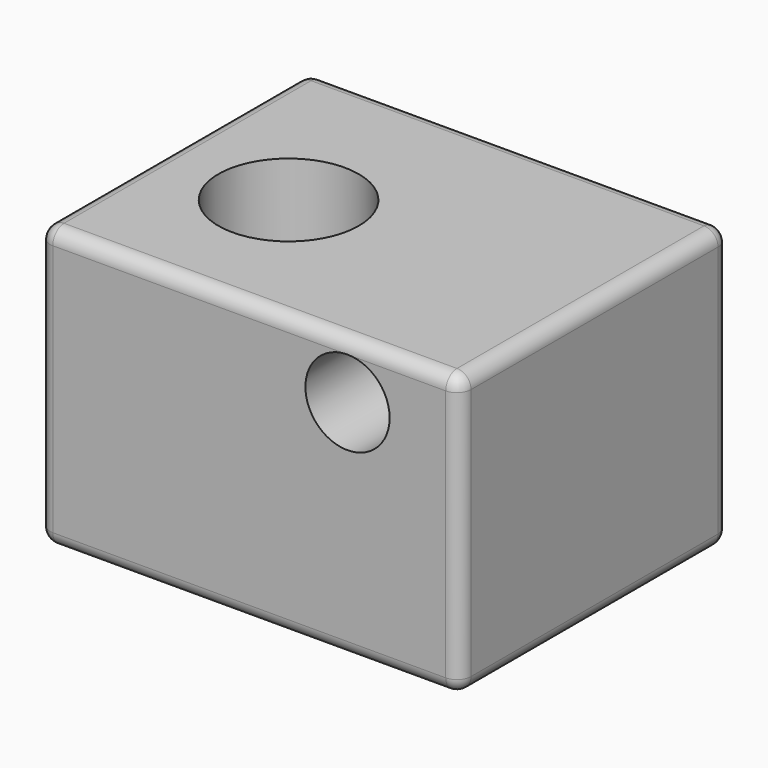
from build123d import *

# Parameters (mm, degrees)
F0_W         = 15
F0_H         = 12
F0_R         = 2.5
F1_DEPTH     = 5
F2_R         = 1.5
F3_DEPTH     = 12.001
F4_R         = 0.49999
F5_T1_DEPTH  = 9.5
F5_T3_DEPTH  = 11
F5_T5_DEPTH  = 14
F5_T8_ANGLE  = 90
F5_T10_ANGLE = 90
F5_T12_ANGLE = 90
F5_T14_ANGLE = 90
F5_S17_W     = 0.5
F5_S17_H     = 0.5
F5_T18_DEPTH = 0.5
F5_S23_W     = 0.5
F5_S23_H     = 0.5
F5_T24_DEPTH = 0.5
F5_S29_W     = 0.5
F5_S29_H     = 0.5
F5_T30_DEPTH = 0.5
F5_S35_W     = 0.5
F5_S35_H     = 0.5
F5_T36_DEPTH = 0.5


# Not quite as in the source:
# - a fillet or chamfer that OpenCascade refuses, or shapes differently, is made with other operations: its cross-section is extruded or revolved along the edge and cut away or added
# - a fillet or chamfer is up to 0.001 mm smaller than in the source, because OpenCascade refuses the exact size


with BuildPart() as f1:
    # F0 (on Top) → F1 (new body, symmetric)
    with BuildSketch(Plane.XY):
        with Locations((7.5, 6)):
            Rectangle(F0_W, F0_H)
        with Locations((4.5, 5.5)):
            Circle(F0_R, mode=Mode.SUBTRACT)
    extrude(amount=F1_DEPTH, both=True)

    # F2 (on face) → F3 (cut, through all)
    with BuildSketch(Plane.XZ):
        with Locations((11, 3)):
            Circle(F2_R)
    extrude(amount=-F3_DEPTH, mode=Mode.SUBTRACT)

    # F4 (radius 0.5 in the source; OpenCascade refuses exactly that, so slightly less here)
    f4_edges = [f1.edges().sort_by_distance(p)[0] for p in [
        (7.5, 0, 5),
        (15, 6, 5),
        (7.5, 12, 5),
        (0, 6, 5),
    ]]
    fillet(f4_edges, radius=F4_R)

    # F5: fillet of radius 0.5 on 8 edges, made by hand

    # F5_s2 → F5_t1 (cut)
    with BuildSketch(Plane.XY.offset(-4.5)):
        with BuildLine():
            ThreePointArc((14.5, 0), (14.8535533906, 0.1464466094), (15, 0.5))
            Line((15, 0.5), (15, 0))
            Line((15, 0), (14.5, 0))
        make_face()
        with BuildLine():
            ThreePointArc((0, 0.5), (0.1464466094, 0.1464466094), (0.5, 0))
            Line((0.5, 0), (0, 0))
            Line((0, 0), (0, 0.5))
        make_face()
        with BuildLine():
            ThreePointArc((0, 11.5), (0.1464466094, 11.8535533906), (0.5, 12))
            Line((0.5, 12), (0, 12))
            Line((0, 12), (0, 11.5))
        make_face()
        with BuildLine():
            ThreePointArc((14.5, 12), (14.8535533906, 11.8535533906), (15, 11.5))
            Line((15, 11.5), (15, 12))
            Line((15, 12), (14.5, 12))
        make_face()
    extrude(amount=F5_T1_DEPTH, mode=Mode.SUBTRACT)

    # F5_s4 → F5_t3 (cut)
    with BuildSketch(Plane.XZ.offset(-11.5)):
        with BuildLine():
            ThreePointArc((0, -4.5), (0.1464466094, -4.8535533906), (0.5, -5))
            Line((0.5, -5), (0, -5))
            Line((0, -5), (0, -4.5))
        make_face()
        with BuildLine():
            ThreePointArc((14.5, -5), (14.8535533906, -4.8535533906), (15, -4.5))
            Line((15, -4.5), (15, -5))
            Line((15, -5), (14.5, -5))
        make_face()
    extrude(amount=F5_T3_DEPTH, mode=Mode.SUBTRACT)

    # F5_s6 → F5_t5 (cut)
    with BuildSketch(Plane.YZ.offset(0.5)):
        with BuildLine():
            ThreePointArc((11.5, -5), (11.8535533906, -4.8535533906), (12, -4.5))
            Line((12, -4.5), (12, -5))
            Line((12, -5), (11.5, -5))
        make_face()
        with BuildLine():
            ThreePointArc((0, -4.5), (0.1464466094, -4.8535533906), (0.5, -5))
            Line((0.5, -5), (0, -5))
            Line((0, -5), (0, -4.5))
        make_face()
    extrude(amount=F5_T5_DEPTH, mode=Mode.SUBTRACT)

    # F5_s7 → F5_t8 (revolve, cut)
    with BuildSketch(Plane.XZ.offset(-11.5)):
        with BuildLine():
            ThreePointArc((14.50001, 5), (14.8535563195, 4.8535563195), (15, 4.50001))
            Line((15, 4.50001), (15, 5))
            Line((15, 5), (14.50001, 5))
        make_face()
    revolve(axis=Axis((14.5, 11.5, 5), (0, 0, 1)), revolution_arc=F5_T8_ANGLE, mode=Mode.SUBTRACT)

    # F5_s9 → F5_t10 (revolve, cut)
    with BuildSketch(Plane.YZ.offset(0.5)):
        with BuildLine():
            ThreePointArc((11.50001, 5), (11.8535563195, 4.8535563195), (12, 4.50001))
            Line((12, 4.50001), (12, 5))
            Line((12, 5), (11.50001, 5))
        make_face()
    revolve(axis=Axis((0.5, 11.5, 5), (0, 0, 1)), revolution_arc=F5_T10_ANGLE, mode=Mode.SUBTRACT)

    # F5_s11 → F5_t12 (revolve, cut)
    with BuildSketch(Plane.XZ.offset(-0.5)):
        with BuildLine():
            ThreePointArc((0.49999, 5), (0.1464436805, 4.8535563195), (0, 4.50001))
            Line((0, 4.50001), (0, 5))
            Line((0, 5), (0.49999, 5))
        make_face()
    revolve(axis=Axis((0.5, 0.5, 5), (0, 0, 1)), revolution_arc=F5_T12_ANGLE, mode=Mode.SUBTRACT)

    # F5_s13 → F5_t14 (revolve, cut)
    with BuildSketch(Plane.YZ.offset(14.5)):
        with BuildLine():
            ThreePointArc((0.49999, 5), (0.1464436805, 4.8535563195), (0, 4.50001))
            Line((0, 4.50001), (0, 5))
            Line((0, 5), (0.49999, 5))
        make_face()
    revolve(axis=Axis((14.5, 0.5, 5), (0, 0, 1)), revolution_arc=F5_T14_ANGLE, mode=Mode.SUBTRACT)


with BuildPart() as f5_tool16:
    # F5_s17 → F5_t18 (new body)
    with BuildSketch(Plane.XZ.offset(-0.5)):
        with Locations((14.75, -4.75)):
            Rectangle(F5_S17_W, F5_S17_H)
    extrude(amount=F5_T18_DEPTH)

    # F5_s19 → F5_t20 (revolve, cut)
    with BuildSketch(Plane(origin=(14.5, 0.5, -4.5), x_dir=(-0.7071067812, 0, 0.7071067812), z_dir=(0.7071067812, 0, 0.7071067812))):
        with BuildLine():
            ThreePointArc((0, -0.5), (0.5, 0), (0, 0.5))
            Line((0, 0.5), (0, -0.5))
        make_face()
    revolve(axis=Axis((14.5, 0.5, -4.5), (0, -1, 0)), mode=Mode.SUBTRACT)


with BuildPart() as f1_1:
    add(f1.part)

    # F5_t15: cut F5_tool16
    add(f5_tool16.part, mode=Mode.SUBTRACT)


with BuildPart() as f5_tool22:
    # F5_s23 → F5_t24 (new body)
    with BuildSketch(Plane.YZ.offset(0.5)):
        with Locations((0.25, -4.75)):
            Rectangle(F5_S23_W, F5_S23_H)
    extrude(amount=-F5_T24_DEPTH)

    # F5_s25 → F5_t26 (revolve, cut)
    with BuildSketch(Plane(origin=(0.5, 0.5, -4.5), x_dir=(0, 0.7071067812, 0.7071067812), z_dir=(0, -0.7071067812, 0.7071067812))):
        with BuildLine():
            ThreePointArc((0, -0.5), (0.5, 0), (0, 0.5))
            Line((0, 0.5), (0, -0.5))
        make_face()
    revolve(axis=Axis((0.5, 0.5, -4.5), (-1, 0, 0)), mode=Mode.SUBTRACT)


with BuildPart() as f1_2:
    add(f1_1.part)

    # F5_t21: cut F5_tool22
    add(f5_tool22.part, mode=Mode.SUBTRACT)


with BuildPart() as f5_tool28:
    # F5_s29 → F5_t30 (new body)
    with BuildSketch(Plane.YZ.offset(0.5)):
        with Locations((11.75, -4.75)):
            Rectangle(F5_S29_W, F5_S29_H)
    extrude(amount=-F5_T30_DEPTH)

    # F5_s31 → F5_t32 (revolve, cut)
    with BuildSketch(Plane(origin=(0.5, 11.5, -4.5), x_dir=(0, -0.7071067812, 0.7071067812), z_dir=(0, -0.7071067812, -0.7071067812))):
        with BuildLine():
            ThreePointArc((0, -0.5), (0.5, 0), (0, 0.5))
            Line((0, 0.5), (0, -0.5))
        make_face()
    revolve(axis=Axis((0.5, 11.5, -4.5), (-1, 0, 0)), mode=Mode.SUBTRACT)


with BuildPart() as f1_3:
    add(f1_2.part)

    # F5_t27: cut F5_tool28
    add(f5_tool28.part, mode=Mode.SUBTRACT)


with BuildPart() as f5_tool34:
    # F5_s35 → F5_t36 (new body)
    with BuildSketch(Plane.XY.offset(-4.5)):
        with Locations((14.75, 11.75)):
            Rectangle(F5_S35_W, F5_S35_H)
    extrude(amount=-F5_T36_DEPTH)

    # F5_s37 → F5_t38 (revolve, cut)
    with BuildSketch(Plane(origin=(14.5, 11.5, -4.5), x_dir=(-0.7071067812, -0.7071067812, 0), z_dir=(0.7071067812, -0.7071067812, 0))):
        with BuildLine():
            ThreePointArc((0, -0.5), (0.5, 0), (0, 0.5))
            Line((0, 0.5), (0, -0.5))
        make_face()
    revolve(axis=Axis((14.5, 11.5, -4.5), (0, 0, -1)), mode=Mode.SUBTRACT)


with BuildPart() as f1_4:
    add(f1_3.part)

    # F5_t33: cut F5_tool34
    add(f5_tool34.part, mode=Mode.SUBTRACT)


solid = f1_4.part
